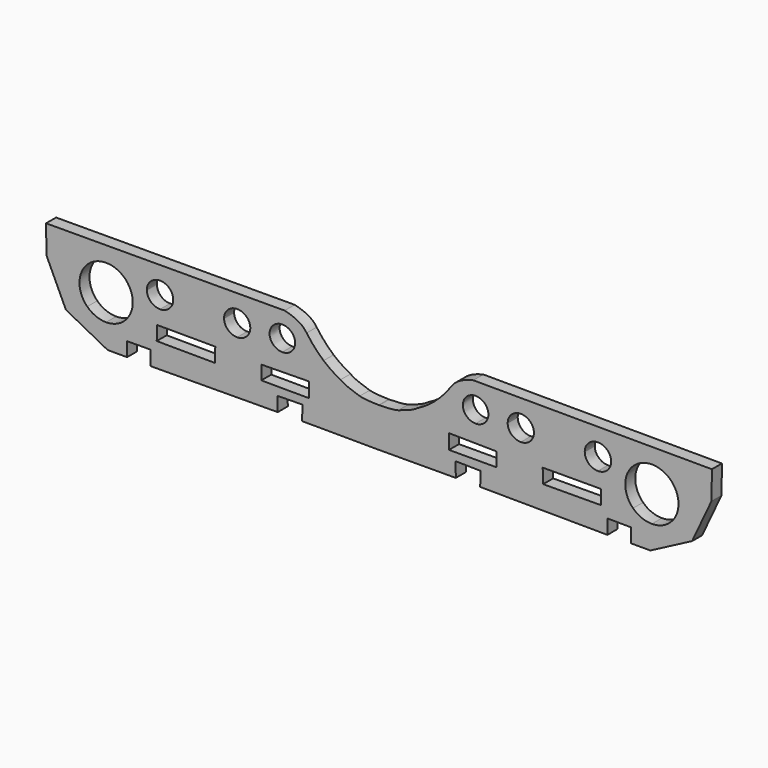
from build123d import *

# Parameters (mm, degrees)
F1_DEPTH = 4


# Not quite as in the source:
# - ends of sketch curves that miss each other by under 0.0002 mm in the source are joined


with BuildPart() as f1:
    # F0 (on Front) → F1 (new body)
    with BuildSketch(Plane.XZ):
        with BuildLine():
            Line((106.284643934, 13.8998607662), (30.113878934, 14.1357487662))
            add(Edge.make_bspline(
                [(23.098041934, 10.1267067662), (24.668698934, 12.4514187662), (27.213718934, 13.4064397662), (30.113878934, 14.1357487662)],
                knots=[0, 0, 0, 0, 1, 1, 1, 1], degree=3))
            add(Edge.make_bspline(
                [(17.685838934, 4.1131437662), (19.766398934, 5.9102937662), (21.551885934, 7.9287527662), (23.098041934, 10.1267067662)],
                knots=[0, 0, 0, 0, 1, 1, 1, 1], degree=3))
            add(Edge.make_bspline(
                [(12.273635934, 0.5050027662), (14.367411934, 1.5628647662), (16.125785934, 2.7884227662), (17.685838934, 4.1131437662)],
                knots=[0, 0, 0, 0, 1, 1, 1, 1], degree=3))
            add(Edge.make_bspline(
                [(6.159823934, -2.1008732338), (8.205815934, -1.2725192338), (10.346098934, -0.9156272338), (12.273635934, 0.5050027662)],
                knots=[0, 0, 0, 0, 1, 1, 1, 1], degree=3))
            add(Edge.make_bspline(
                [(0.096170934, -2.6521172338), (2.268275934, -2.6192522338), (4.383741934, -2.5297572338), (6.159823934, -2.1008732338)],
                knots=[0, 0, 0, 0, 1, 1, 1, 1], degree=3))
            Line((0.096170934, -2.6521172338), (0, -2.6521172338))
            Line((0, -2.6521172338), (0, -15.2320805937))
            Line((0, -15.2320805937), (24.524526934, -15.1302652338))
            Line((24.524526934, -15.1302652338), (24.465801934, -10.4545552338))
            Line((24.465801934, -10.4545552338), (32.372008934, -10.5730212338))
            Line((32.372008934, -10.5730212338), (32.318833934, -15.1302652338))
            Line((32.318833934, -15.1302652338), (72.927583934, -15.4015902338))
            Line((72.927583934, -15.4015902338), (72.987358934, -10.7668702338))
            Line((72.987358934, -10.7668702338), (80.404101934, -10.8266232338))
            Line((80.404101934, -10.8266232338), (80.427351934, -15.3307162338))
            Line((80.427351934, -15.3307162338), (86.641378934, -15.3307162338))
            Line((86.641378934, -15.3307162338), (99.965361934, -8.3503262338))
            Line((99.965361934, -8.3503262338), (106.167223934, 4.9149507662))
            Line((106.167223934, 4.9149507662), (106.284643934, 13.8998607662))
        make_face()
        Polygon((22.346346934, -7.9641002338), (22.396461934, -3.2534742338), (37.580713934, -3.4539262338), (37.580705934, -7.9139852338), align=None, mode=Mode.SUBTRACT)
        Polygon((52.414160934, -7.8137592338), (52.263830934, -3.2033612338), (70.905883934, -3.1532462338), (70.955983934, -7.7135322338), align=None, mode=Mode.SUBTRACT)
        with BuildLine():
            add(Edge.make_bspline(
                [(30.851675934, 9.9924447662), (33.101845934, 9.9924437662), (34.925968934, 8.2476447662), (34.925968934, 6.0953267662)],
                knots=[0, 0, 0, 0, 1, 1, 1, 1], degree=3))
            add(Edge.make_bspline(
                [(34.925968934, 6.0953267662), (34.925968934, 3.9430077662), (33.101845934, 2.1982097662), (30.851675934, 2.1982087662)],
                knots=[0, 0, 0, 0, 1, 1, 1, 1], degree=3))
            add(Edge.make_bspline(
                [(30.851675934, 2.1982087662), (28.601506934, 2.1982097662), (26.777383934, 3.9430077662), (26.777383934, 6.0953267662)],
                knots=[0, 0, 0, 0, 1, 1, 1, 1], degree=3))
            add(Edge.make_bspline(
                [(26.777383934, 6.0953267662), (26.777383934, 8.2476447662), (28.601506934, 9.9924437662), (30.851675934, 9.9924447662)],
                knots=[0, 0, 0, 0, 1, 1, 1, 1], degree=3))
        make_face(mode=Mode.SUBTRACT)
        with BuildLine():
            add(Edge.make_bspline(
                [(45.273838934, 9.6413387662), (47.584508934, 9.6413367662), (49.457676934, 7.8633577662), (49.457675934, 5.6701097662)],
                knots=[0, 0, 0, 0, 1, 1, 1, 1], degree=3))
            add(Edge.make_bspline(
                [(49.457675934, 5.6701097662), (49.457676934, 3.4768617662), (47.584508934, 1.6988817662), (45.273838934, 1.6988807662)],
                knots=[0, 0, 0, 0, 1, 1, 1, 1], degree=3))
            add(Edge.make_bspline(
                [(45.273838934, 1.6988807662), (42.963168934, 1.6988817662), (41.090000934, 3.4768617662), (41.090001934, 5.6701097662)],
                knots=[0, 0, 0, 0, 1, 1, 1, 1], degree=3))
            add(Edge.make_bspline(
                [(41.090001934, 5.6701097662), (41.090000934, 7.8633577662), (42.963168934, 9.6413367662), (45.273838934, 9.6413387662)],
                knots=[0, 0, 0, 0, 1, 1, 1, 1], degree=3))
        make_face(mode=Mode.SUBTRACT)
        with BuildLine():
            add(Edge.make_bspline(
                [(69.901340934, 9.6329967662), (72.226976934, 9.6329957662), (74.112275934, 7.8270207662), (74.112275934, 5.5992367662)],
                knots=[0, 0, 0, 0, 1, 1, 1, 1], degree=3))
            add(Edge.make_bspline(
                [(74.112275934, 5.5992367662), (74.112276934, 3.3714527662), (72.226976934, 1.5654767662), (69.901340934, 1.5654757662)],
                knots=[0, 0, 0, 0, 1, 1, 1, 1], degree=3))
            add(Edge.make_bspline(
                [(69.901340934, 1.5654757662), (67.575705934, 1.5654767662), (65.690405934, 3.3714527662), (65.690405934, 5.5992367662)],
                knots=[0, 0, 0, 0, 1, 1, 1, 1], degree=3))
            add(Edge.make_bspline(
                [(65.690405934, 5.5992367662), (65.690406934, 7.8270207662), (67.575705934, 9.6329957662), (69.901340934, 9.6329967662)],
                knots=[0, 0, 0, 0, 1, 1, 1, 1], degree=3))
        make_face(mode=Mode.SUBTRACT)
        with BuildLine():
            add(Edge.make_bspline(
                [(93.135414934, 6.5860497662), (94.730039934, 5.0180057662), (95.625890934, 2.8912817662), (95.625890934, 0.6737337662)],
                knots=[0, 0, 0, 0, 1, 1, 1, 1], degree=3))
            add(Edge.make_bspline(
                [(95.625890934, 0.6737337662), (95.625890934, -1.5438152338), (94.730039934, -3.6705392338), (93.135413934, -5.2385832338)],
                knots=[0, 0, 0, 0, 1, 1, 1, 1], degree=3))
            add(Edge.make_bspline(
                [(93.135413934, -5.2385832338), (91.540788934, -6.8066262338), (89.378011934, -7.6875442338), (87.122871934, -7.6875432338)],
                knots=[0, 0, 0, 0, 1, 1, 1, 1], degree=3))
            add(Edge.make_bspline(
                [(87.122871934, -7.6875432338), (84.867730934, -7.6875442338), (82.704953934, -6.8066262338), (81.110328934, -5.2385832338)],
                knots=[0, 0, 0, 0, 1, 1, 1, 1], degree=3))
            add(Edge.make_bspline(
                [(81.110328934, -5.2385832338), (79.515702934, -3.6705392338), (78.619851934, -1.5438152338), (78.619851934, 0.6737337662)],
                knots=[0, 0, 0, 0, 1, 1, 1, 1], degree=3))
            add(Edge.make_bspline(
                [(78.619851934, 0.6737337662), (78.619851934, 2.8912817662), (79.515702934, 5.0180057662), (81.110327934, 6.5860497662)],
                knots=[0, 0, 0, 0, 1, 1, 1, 1], degree=3))
            add(Edge.make_bspline(
                [(81.110327934, 6.5860497662), (82.704953934, 8.1540937662), (84.867730934, 9.0350107662), (87.122871934, 9.0350107662)],
                knots=[0, 0, 0, 0, 1, 1, 1, 1], degree=3))
            add(Edge.make_bspline(
                [(87.122871934, 9.0350107662), (89.378011934, 9.0350107662), (91.540788934, 8.1540937662), (93.135414934, 6.5860497662)],
                knots=[0, 0, 0, 0, 1, 1, 1, 1], degree=3))
        make_face(mode=Mode.SUBTRACT)
    extrude(amount=F1_DEPTH)

    # F2: F1 across plane


with BuildPart() as f1_1:
    add(f1.part)
    add(f1.part.mirror(Plane.YZ))


solid = f1_1.part
